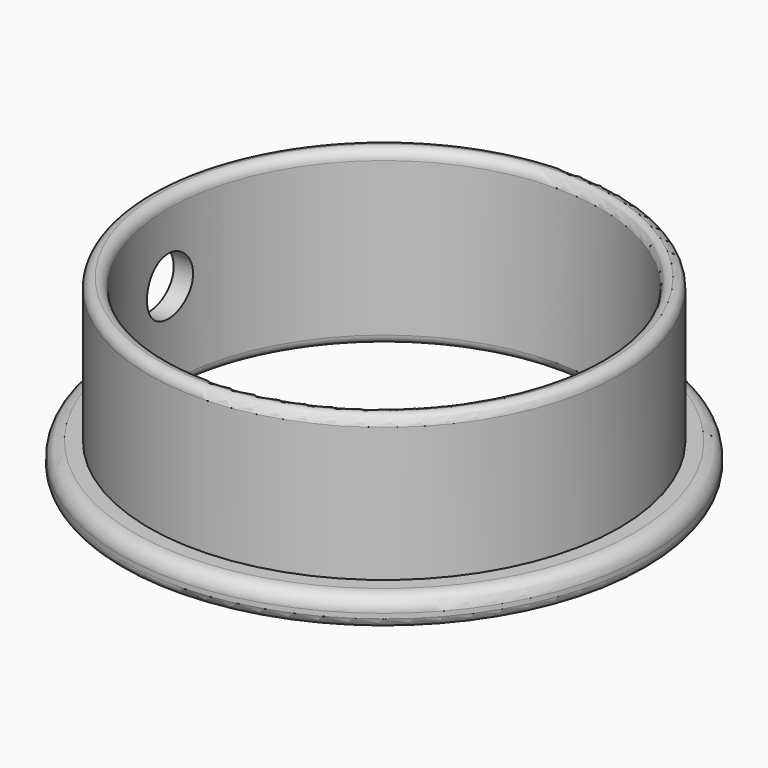
from build123d import *

# Parameters (mm, degrees)
F0_R     = 27.5
F0_R_2   = 24.5
F1_DEPTH = 3
F0_R_3   = 22.5
F2_DEPTH = 18
F3_R     = 1
F4_R     = 1.5
F5_R     = 0.99999
F7_D     = 6
F7_DEPTH = 25
F7_TIP   = 1.8025818571


# Not quite as in the source:
# - a fillet or chamfer is up to 0.001 mm smaller than in the source, because OpenCascade refuses the exact size


with BuildPart() as f1:
    # F0 (on Top) → F1 (new body)
    with BuildSketch(Plane.XY):
        Circle(F0_R)
        Circle(F0_R_2, mode=Mode.SUBTRACT)
    extrude(amount=F1_DEPTH)

    # F0 (on Top) → F2 (join)
    with BuildSketch(Plane.XY):
        Circle(F0_R_2)
        Circle(F0_R_3, mode=Mode.SUBTRACT)
    extrude(amount=F2_DEPTH)

    # F3
    f3_edges = [f1.edges().sort_by_distance(p)[0] for p in [
        (-27.5, 0, 0),
        (-22.5, 0, 0),
    ]]
    fillet(f3_edges, radius=F3_R)

    # F4
    f4_edges = [f1.edges().sort_by_distance(p)[0] for p in [
        (-27.5, 0, 3),
    ]]
    fillet(f4_edges, radius=F4_R)

    # F5 (radius 1 in the source; OpenCascade refuses exactly that, so slightly less here)
    f5_edges = [f1.edges().sort_by_distance(p)[0] for p in [
        (-22.5, 0, 18),
        (-24.5, 0, 18),
    ]]
    fillet(f5_edges, radius=F5_R)

    # F7 (one way)
    with BuildSketch(Plane.YZ):
        with Locations((0, 9.8607558757)):
            Circle(F7_D / 2)
    extrude(amount=-F7_DEPTH, mode=Mode.SUBTRACT)
    with Locations(Plane.YZ):
        with Locations((0, 9.8607558757)):
            with Locations((0, 0, -(F7_DEPTH + F7_TIP / 2))):  # 118° drill point
                Cone(0, F7_D / 2, F7_TIP, mode=Mode.SUBTRACT)


solid = f1.part
